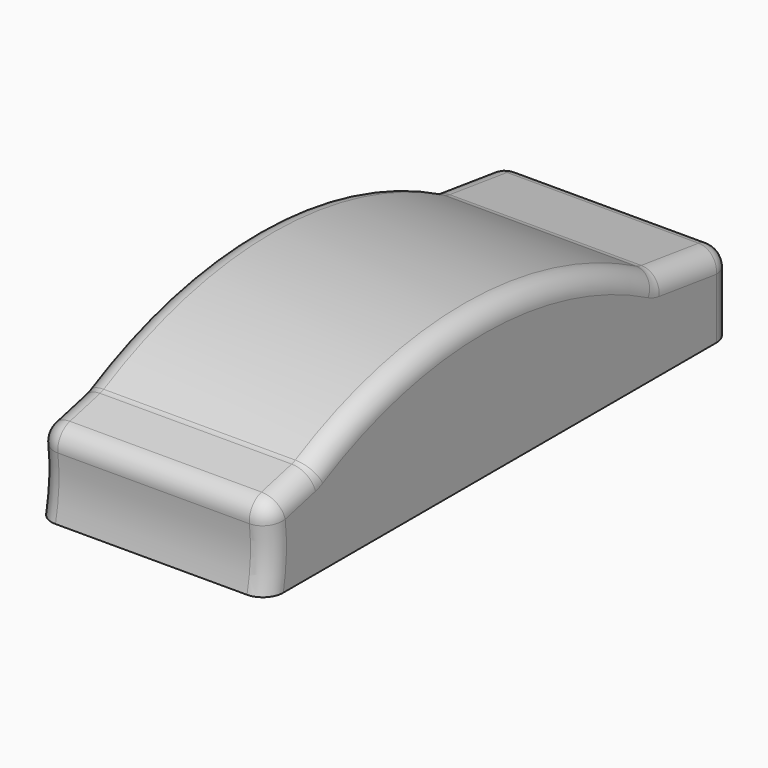
from build123d import *

# Parameters (mm, degrees)
F1_DEPTH = 29
F2_F1_R  = 5
F2_F2_R  = 5
F3_T     = -2.5


with BuildPart() as f1:
    # F0 (on Right) → F1 (new body, symmetric)
    with BuildSketch(Plane.YZ):
        with BuildLine():
            ThreePointArc((-71.5784906799, 19.7169460854), (-70.4874573475, 9.8584730427), (-71.5784906799, 0))
            Line((-71.5784906799, 0), (-54.9704477794, 0))
            ThreePointArc((-54.9704477794, 0), (-43.1382882132, 14), (-31.306128647, 0))
            Line((-31.306128647, 0), (16.2495522206, 0))
            ThreePointArc((16.2495522206, 0), (28.0817117868, 14), (39.913871353, 0))
            Line((39.913871353, 0), (74.2074146826, 0))
            Line((74.2074146826, 0), (74.2074146826, 19.4779538288))
            Line((74.2074146826, 19.4779538288), (51.0250648113, 22.5848669347))
            ThreePointArc((51.0250648113, 22.5848669347), (-2.8965217341, 36.6382547678), (-56.9998987666, 23.3018459996))
            Line((-56.9998987666, 23.3018459996), (-71.5784906799, 19.7169460854))
        make_face()
        with BuildLine():
            ThreePointArc((-31.306128647, 0), (-43.1382882132, 14), (-54.9704477794, 0))
            Line((-54.9704477794, 0), (-31.306128647, 0))
        make_face()
        with BuildLine():
            ThreePointArc((39.913871353, 0), (28.0817117868, 14), (16.2495522206, 0))
            Line((16.2495522206, 0), (39.913871353, 0))
        make_face()
    extrude(amount=F1_DEPTH, both=True)

    # F2: fillet of radius 5 on 10 edges, made by hand

    # F2_f1
    f2_f1_edges = [f1.edges().sort_by_distance(p)[0] for p in [
        (0, -56.9998987666, 23.3018459996),
        (0, 51.0250648113, 22.5848669347),
    ]]
    fillet(f2_f1_edges, radius=F2_F1_R)

    # F2_f2
    f2_f2_edges = [f1.edges().sort_by_distance(p)[0] for p in [
        (0, -71.5784906799, 19.7169460854),
        (-29, -70.4874573475, 9.8584730427),
        (29, -70.4874573475, 9.8584730427),
        (-29, -3.0466412139, 36.6391517316),
        (29, -3.0466412139, 36.6391517316),
        (0, 74.2074146826, 19.4779538288),
        (29, 74.2074146826, 9.7389769144),
        (-29, 74.2074146826, 9.7389769144),
        (29, 51.0608622621, 22.6625045572),
        (29, -57.0196487491, 23.3351165373),
        (-29, 51.0608622621, 22.6625045572),
        (-29, -57.0196487491, 23.3351165373),
    ]]
    fillet(f2_f2_edges, radius=F2_F2_R)

    # F3
    f3_openings = [f1.faces().sort_by_distance(p)[0] for p in [
        (0, 1.316584, 0),
    ]]
    offset(amount=F3_T, openings=f3_openings, kind=Kind.INTERSECTION)


solid = f1.part
